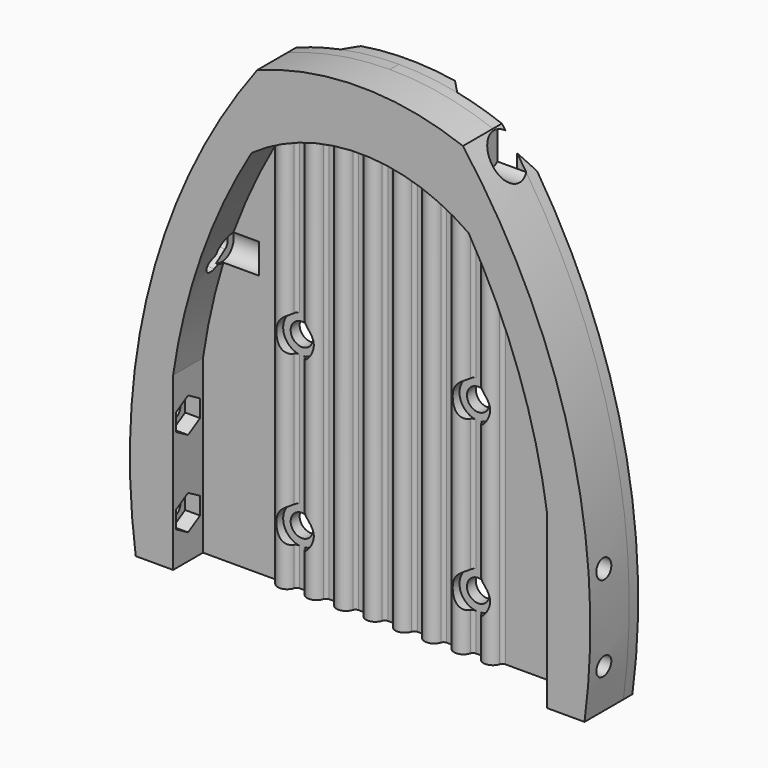
from build123d import *

# Parameters (mm, degrees)
F1_DEPTH       = 3
F3_DEPTH       = 10
F6_R           = 1
F10_R          = 5
F11_DEPTH      = 5
F11_DEPTH_BACK = 25
F12_R          = 5
F13_DEPTH      = 5
F13_DEPTH_BACK = 25
F14_R          = 3
F15_DEPTH      = 25
F16_R          = 5
F17_DEPTH      = 25
F19_DEPTH      = 3
F20_SIZE       = 2.99999
F21_R          = 2.5
F22_DEPTH      = 25
F22_DEPTH_BACK = 111.5543717068
F24_DEPTH      = 4
F26_DEPTH      = 4
F28_DEPTH      = 5.0762168218
F28_DEPTH_BACK = 15
F29_R          = 4
F30_DEPTH      = 10


# Not quite as in the source:
# - a fillet or chamfer is up to 0.001 mm smaller than in the source, because OpenCascade refuses the exact size
# - a feature names something its author has since deleted; it is built from what else it names


with BuildPart() as f1:
    # F0 (on Front) → F1 (new body)
    with BuildSketch(Plane.XZ):
        with BuildLine():
            ThreePointArc((0, 130), (-13.9754248594, 128.7398367266), (-27.5, 125))
            ThreePointArc((-27.5, 125), (-56.0831977608, 65.7066314178), (-60, 0))
            Line((-60, 0), (0, 0))
            Line((0, 0), (60, 0))
            ThreePointArc((60, 0), (56.0831977608, 65.7066314178), (27.5, 125))
            ThreePointArc((27.5, 125), (13.9754248594, 128.7398367266), (0, 130))
        make_face()
    extrude(amount=F1_DEPTH)

    # F2 (on face) → F3 (join)
    with BuildSketch(Plane.XZ.offset(3)):
        with BuildLine():
            ThreePointArc((60, 0), (56.0831977608, 65.7066314178), (27.5, 125))
            ThreePointArc((27.5, 125), (0, 130), (-27.5, 125))
            ThreePointArc((-27.5, 125), (-56.0831977608, 65.7066314178), (-60, 0))
            Line((-60, 0), (-50, 0))
            ThreePointArc((-50, 0), (-51.6504278949, 22.9288766178), (-50, 45.8577532355))
            ThreePointArc((-50, 45.8577532355), (-42.4331694009, 76.4672184834), (-29.0139046296, 105))
            ThreePointArc((-29.0139046296, 105), (0, 114.2790798465), (29.0139046296, 105))
            ThreePointArc((29.0139046296, 105), (42.4331694009, 76.4672184834), (50, 45.8577532355))
            ThreePointArc((50, 45.8577532355), (51.6504278949, 22.9288766178), (50, 0))
            Line((50, 0), (60, 0))
        make_face()
        with BuildLine():
            Line((50, 45.8577532355), (50, 0))
            ThreePointArc((50, 0), (51.6504278949, 22.9288766178), (50, 45.8577532355))
        make_face()
        with BuildLine():
            ThreePointArc((-50, 45.8577532355), (-51.6504278949, 22.9288766178), (-50, 0))
            Line((-50, 0), (-50, 45.8577532355))
        make_face()
    extrude(amount=F3_DEPTH)

    # F4 (on face) → F5 (join, up to the next surface of F1)
    with BuildSketch(Plane(origin=(0, 0, 0), x_dir=(1, 0, 0), z_dir=(0, 0, -1))):
        with BuildLine():
            Line((-30, 3), (-25, 3))
            ThreePointArc((-25, 3), (-27.5, 5.5), (-30, 3))
        make_face()
        with BuildLine():
            Line((-22.1428571429, 3), (-17.1428571429, 3))
            ThreePointArc((-17.1428571429, 3), (-19.6428571429, 5.5), (-22.1428571429, 3))
        make_face()
        with BuildLine():
            Line((-14.2857142857, 3), (-9.2857142857, 3))
            ThreePointArc((-9.2857142857, 3), (-11.7857142857, 5.5), (-14.2857142857, 3))
        make_face()
        with BuildLine():
            Line((-6.4285714286, 3), (-1.4285714286, 3))
            ThreePointArc((-1.4285714286, 3), (-3.9285714286, 5.5), (-6.4285714286, 3))
        make_face()
        with BuildLine():
            Line((1.4285714286, 3), (6.4285714286, 3))
            ThreePointArc((6.4285714286, 3), (3.9285714286, 5.5), (1.4285714286, 3))
        make_face()
        with BuildLine():
            Line((9.2857142857, 3), (14.2857142857, 3))
            ThreePointArc((14.2857142857, 3), (11.7857142857, 5.5), (9.2857142857, 3))
        make_face()
        with BuildLine():
            Line((17.1428571429, 3), (22.1428571429, 3))
            ThreePointArc((22.1428571429, 3), (19.6428571429, 5.5), (17.1428571429, 3))
        make_face()
        with BuildLine():
            Line((25, 3), (30, 3))
            ThreePointArc((30, 3), (27.5, 5.5), (25, 3))
        make_face()
    extrude(until=Until.NEXT, dir=(0, 0, 1))

    # F6
    f6_edges = [f1.edges().sort_by_distance(p)[0] for p in [
        (-30, -3, 51.662692),
        (-25, -3, 53.790175),
        (-17.142857, -3, 55.624229),
        (-9.285714, -3, 56.704635),
        (-1.428571, -3, 57.129334),
        (6.428571, -3, 56.932046),
        (14.285714, -3, 56.097411),
        (22.142857, -3, 54.554345),
        (30, -3, 51.662692),
        (-22.142857, -3, 54.554345),
        (-14.285714, -3, 56.097411),
        (-6.428571, -3, 56.932046),
        (1.428571, -3, 57.129334),
        (9.285714, -3, 56.704635),
        (17.142857, -3, 55.624229),
        (25, -3, 53.790175),
    ]]
    fillet(f6_edges, radius=F6_R)

    # F10 (on offset) → F11 (cut, two sides)
    with BuildSketch(Plane.YZ.offset(31.337)) as f11_sk:
        with Locations((-3, 119.67874604)):
            Circle(F10_R)
    extrude(amount=-F11_DEPTH, mode=Mode.SUBTRACT)
    extrude(f11_sk.sketch, amount=F11_DEPTH_BACK, mode=Mode.SUBTRACT)

    # F12 (on offset) → F13 (cut, two sides)
    with BuildSketch(Plane.YZ.offset(-31.337)) as f13_sk:
        with Locations((-3, 119.67874604)):
            Circle(F12_R)
    extrude(amount=F13_DEPTH, mode=Mode.SUBTRACT)
    extrude(f13_sk.sketch, amount=-F13_DEPTH_BACK, mode=Mode.SUBTRACT)

    # F14 (on face) → F15 (cut)
    with BuildSketch(Plane.XZ.offset(3)):
        with Locations((-23.5714285714, 15)):
            Circle(F14_R)
        with Locations((-23.5714285714, 60)):
            Circle(F14_R)
        with Locations((23.5714285714, 15)):
            Circle(F14_R)
        with Locations((23.5714285714, 60)):
            Circle(F14_R)
    extrude(amount=-F15_DEPTH, mode=Mode.SUBTRACT)

    # F16 (on face) → F17 (cut)
    with BuildSketch(Plane.XZ.offset(3)):
        with Locations((23.5714285714, 60)):
            Circle(F16_R)
        with Locations((-23.5714285714, 60)):
            Circle(F16_R)
        with Locations((-23.5714285714, 15)):
            Circle(F16_R)
        with Locations((23.5714285714, 15)):
            Circle(F16_R)
    extrude(amount=F17_DEPTH, mode=Mode.SUBTRACT)

    # F18 (on face) → F19 (join)
    with BuildSketch(Plane(origin=(0, 0, 0), x_dir=(-1, 0, 0), z_dir=(0, 1, 0))):
        with BuildLine():
            Line((-15.5714285714, 0), (15.5714285714, 0))
            Line((15.5714285714, 0), (15.5714285714, 128.4324701596))
            ThreePointArc((15.5714285714, 128.4324701596), (0, 130), (-15.5714285714, 128.4324701596))
            Line((-15.5714285714, 128.4324701596), (-15.5714285714, 0))
        make_face()
        with BuildLine():
            Line((31.5714285714, 0), (60, 0))
            ThreePointArc((60, 0), (56.9259044213, 62.3233608827), (31.5714285714, 119.3391650928))
            Line((31.5714285714, 119.3391650928), (31.5714285714, 0))
        make_face()
        with BuildLine():
            ThreePointArc((-31.5714285714, 119.3391650928), (-56.9259044213, 62.3233608827), (-60, 0))
            Line((-60, 0), (-31.5714285714, 0))
            Line((-31.5714285714, 0), (-31.5714285714, 119.3391650928))
        make_face()
    extrude(amount=F19_DEPTH)

    # F20 (size 3 in the source; OpenCascade refuses exactly that, so slightly less here)
    f20_edges = [f1.edges().sort_by_distance(p)[0] for p in [
        (-15.571429, 3, 64.216235),
        (15.571429, 3, 64.216235),
        (31.571429, 3, 59.669583),
        (-31.571429, 3, 59.669583),
        (0, 3, 0),
    ]]
    chamfer(f20_edges, length=F20_SIZE)

    # F21 (on face) → F22 (cut, two sides)
    with BuildSketch(Plane.YZ.offset(-50)) as f22_sk:
        with Locations((-8, 11.4644383089)):
            Circle(F21_R)
        with Locations((-8, 34.3933149266)):
            Circle(F21_R)
    extrude(amount=-F22_DEPTH, mode=Mode.SUBTRACT)
    extrude(f22_sk.sketch, amount=F22_DEPTH_BACK, mode=Mode.SUBTRACT)

    # F23 (on face) → F24 (cut)
    with BuildSketch(Plane.YZ.offset(-50)):
        Polygon((-8, 16.1121079759), (-12.025, 13.7882731424), (-12.025, 9.1406034754), (-8, 6.8167686419), (-3.975, 9.1406034754), (-3.975, 13.7882731424), align=None)
        Polygon((-8, 39.0409845936), (-12.025, 36.7171497601), (-12.025, 32.0694800932), (-8, 29.7456452597), (-3.975, 32.0694800932), (-3.975, 36.7171497601), align=None)
    extrude(amount=-F24_DEPTH, mode=Mode.SUBTRACT)

    # F25 (on face) → F26 (cut)
    with BuildSketch(Plane(origin=(50, 0, 0), x_dir=(0, -1, 0), z_dir=(-1, 0, 0))):
        Polygon((12.025, 32.0694800932), (12.025, 36.7171497601), (8, 39.0409845936), (3.975, 36.7171497601), (3.975, 32.0694800932), (8, 29.7456452597), align=None)
        Polygon((12.025, 9.1406034754), (12.025, 13.7882731424), (8, 16.1121079759), (3.975, 13.7882731424), (3.975, 9.1406034754), (8, 6.8167686419), align=None)
    extrude(amount=-F26_DEPTH, mode=Mode.SUBTRACT)

    # F27 (on face) → F28 (cut, two sides)
    with BuildSketch(Plane.YZ.offset(-50)) as f28_sk:
        with BuildLine():
            ThreePointArc((-1.8528471273, 72.6407757579), (-1.3616959114, 75.4262327192), (-4.1471528727, 75.9173839351))
            Line((-4.1471528727, 75.9173839351), (-8.2429130941, 73.0495017533))
            ThreePointArc((-8.2429130941, 73.0495017533), (-8.73406431, 70.2640447921), (-5.9486073487, 69.7728935762))
            Line((-5.9486073487, 69.7728935762), (-1.8528471273, 72.6407757579))
        make_face()
    extrude(amount=-F28_DEPTH, mode=Mode.SUBTRACT)
    extrude(f28_sk.sketch, amount=F28_DEPTH_BACK, mode=Mode.SUBTRACT)

    # F29 (on face) → F30 (cut)
    with BuildSketch(Plane(origin=(-35, 0, 0), x_dir=(0, -1, 0), z_dir=(-1, 0, 0))):
        with Locations((3, 74.0583052578)):
            Circle(F29_R)
    extrude(amount=F30_DEPTH, mode=Mode.SUBTRACT)


solid = f1.part
